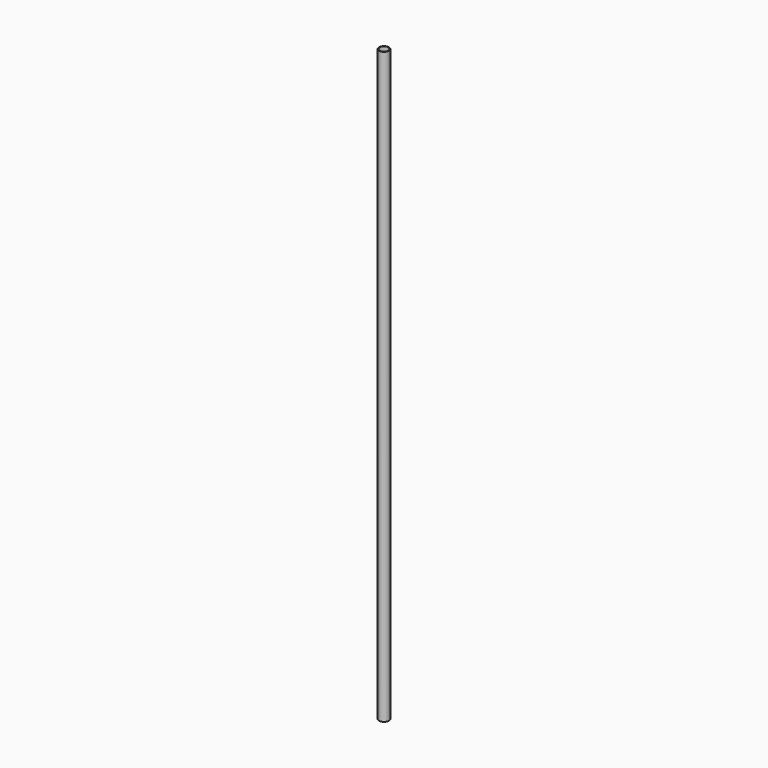
from build123d import *

# Parameters (mm, degrees)
F0_R     = 20
F0_R_2   = 18
F1_DEPTH = 2400
F3_D     = 8
F3_DEPTH = 20.001
F5_D     = 8
F5_DEPTH = 20.0010001


# Not quite as in the source:
# - a feature names something its author has since deleted; it is built from what else it names


with BuildPart() as f1:
    # F0 (on Top) → F1 (new body)
    with BuildSketch(Plane.XY):
        Circle(F0_R)
        Circle(F0_R_2, mode=Mode.SUBTRACT)
    extrude(amount=F1_DEPTH)

    # F3 (through all, one way)
    with BuildSketch(Plane.XZ):
        with Locations((0, 1800), (9.0000000782, 1206.2214374542), (0, 1000), (-13.0000011995, 1400), (0, 2200), (-13.0000011995, 1600), (4.9999998882, 2000)):
            Circle(F3_D / 2)
    extrude(amount=-F3_DEPTH, mode=Mode.SUBTRACT)

    # F5 (through all, one way)
    with BuildSketch(Plane.YZ):
        with Locations((-10.0234504789, 1501.0036230087), (0, 1100), (0, 1300), (0, 1900), (-10.0234504789, 1701.0036230087), (0, 2300), (0, 2100)):
            Circle(F5_D / 2)
    extrude(amount=-F5_DEPTH, mode=Mode.SUBTRACT)


solid = f1.part
